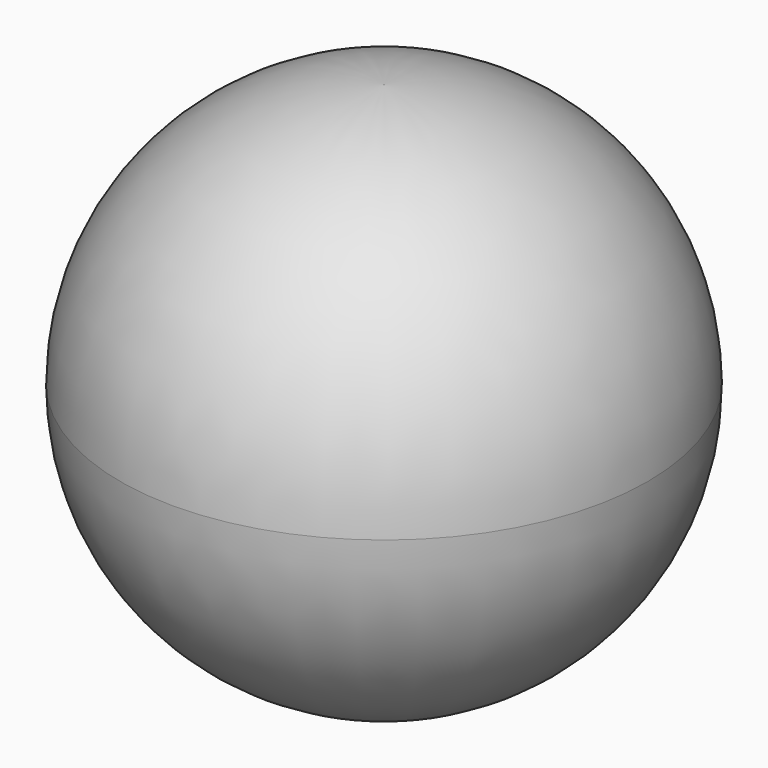
from build123d import *

# Parameters (mm, degrees)
F0_R     = 38.1718882339
F1_DEPTH = 76.2
F2_R     = 38.09999


# Not quite as in the source:
# - a fillet or chamfer is up to 0.001 mm smaller than in the source, because OpenCascade refuses the exact size


with BuildPart() as f1:
    # F0 (on Top) → F1 (new body)
    with BuildSketch(Plane.XY):
        Circle(F0_R)
    extrude(amount=-F1_DEPTH)

    # F2 (radius 38.1 in the source; OpenCascade refuses exactly that, so slightly less here)
    f2_edges = [f1.edges().sort_by_distance(p)[0] for p in [
        (-38.171888, 0, 0),
        (-38.171888, 0, -76.2),
    ]]
    fillet(f2_edges, radius=F2_R)


solid = f1.part
